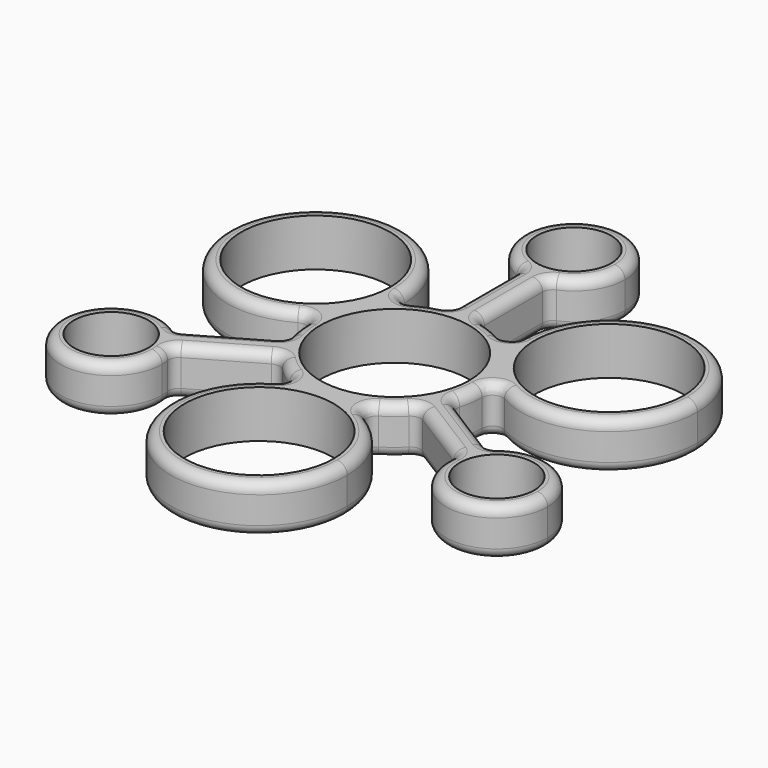
from build123d import *

# Parameters (mm, degrees)
F0_R     = 5.5
F0_R_2   = 11
F1_DEPTH = 7
F2_F1_R  = 1.5
F2_F2_R  = 1.5


with BuildPart() as f1:
    # F0 (on Top) → F1 (new body)
    with BuildSketch(Plane.XY):
        with BuildLine():
            ThreePointArc((2, 25.8452325787), (5.9686681932, 28.5321731949), (7.5, 33.0736487261))
            ThreePointArc((7.5, 33.0736487261), (-4.5414755311, 39.0423169192), (-2, 25.8452325787))
            ThreePointArc((-2, 25.8452325787), (0, 25.5736487261), (2, 25.8452325787))
        make_face()
        with Locations((0, 33.0736487261)):
            Circle(F0_R, mode=Mode.SUBTRACT)
        with BuildLine():
            ThreePointArc((2, 25.8452325787), (0, 25.5736487261), (-2, 25.8452325787))
            Line((-2, 25.8452325787), (-2, 12.8452325787))
            ThreePointArc((-2, 12.8452325787), (0, 13), (2, 12.8452325787))
            Line((2, 12.8452325787), (2, 25.8452325787))
        make_face()
        with BuildLine():
            ThreePointArc((2, 12.8452325787), (0, 13), (-2, 12.8452325787))
            ThreePointArc((-2, 12.8452325787), (-5.7911798985, 11.6388244846), (-9.0399604402, 9.3423292192))
            ThreePointArc((-9.0399604402, 9.3423292192), (-10.3923048454, 6), (-12.6106746544, 3.1576707808))
            ThreePointArc((-12.6106746544, 3.1576707808), (-12.9751076231, -0.8041033323), (-12.1242977306, -4.6905654818))
            ThreePointArc((-12.1242977306, -4.6905654818), (-11.2583302492, -6.5), (-10.1242977306, -8.1546670969))
            ThreePointArc((-10.1242977306, -8.1546670969), (-7.1839277246, -10.8347211523), (-3.5707142143, -12.5))
            ThreePointArc((-3.5707142143, -12.5), (0, -12), (3.5707142143, -12.5))
            ThreePointArc((3.5707142143, -12.5), (7.1839277246, -10.8347211523), (10.1242977306, -8.1546670969))
            ThreePointArc((10.1242977306, -8.1546670969), (11.2590153555, -6.4988132165), (12.1252863318, -4.6880093186))
            ThreePointArc((12.1252863318, -4.6880093186), (12.7794507377, -2.3844577671), (13, 0))
            ThreePointArc((13, 0), (12.9023015487, 1.5907906041), (12.6106746544, 3.1576707808))
            ThreePointArc((12.6106746544, 3.1576707808), (10.3923048454, 6), (9.0399604402, 9.3423292192))
            ThreePointArc((9.0399604402, 9.3423292192), (5.7911798985, 11.6388244846), (2, 12.8452325787))
        make_face()
        Circle(F0_R_2, mode=Mode.SUBTRACT)
        with BuildLine():
            ThreePointArc((-12.6106746544, 3.1576707808), (-10.3923048454, 6), (-9.0399604402, 9.3423292192))
            ThreePointArc((-9.0399604402, 9.3423292192), (-11.2583302492, 6.5), (-12.6106746544, 3.1576707808))
        make_face()
        with BuildLine():
            ThreePointArc((-12.6106746544, 3.1576707808), (-11.2583302492, 6.5), (-9.0399604402, 9.3423292192))
            ThreePointArc((-9.0399604402, 9.3423292192), (-8.7483335459, 10.9092093959), (-8.6506350946, 12.5))
            ThreePointArc((-8.6506350946, 12.5), (-33.6197513051, 17.5734856991), (-12.6106746544, 3.1576707808))
        make_face()
        with Locations((-21.6506350946, 12.5)):
            Circle(F0_R_2, mode=Mode.SUBTRACT)
        with BuildLine():
            ThreePointArc((34.6506350946, 12.5), (20.0598444905, 25.4023015487), (9.0399604402, 9.3423292192))
            ThreePointArc((9.0399604402, 9.3423292192), (11.2583302492, 6.5), (12.6106746544, 3.1576707808))
            ThreePointArc((12.6106746544, 3.1576707808), (26.7241207937, 0.5308837895), (34.6506350946, 12.5))
        make_face()
        with Locations((21.6506350946, 12.5)):
            Circle(F0_R_2, mode=Mode.SUBTRACT)
        with BuildLine():
            ThreePointArc((12.6106746544, 3.1576707808), (11.2583302492, 6.5), (9.0399604402, 9.3423292192))
            ThreePointArc((9.0399604402, 9.3423292192), (10.3923048454, 6), (12.6106746544, 3.1576707808))
        make_face()
        with BuildLine():
            ThreePointArc((-10.1242977306, -8.1546670969), (-11.2583302492, -6.5), (-12.1242977306, -4.6905654818))
            Line((-12.1242977306, -4.6905654818), (-23.3826279798, -11.1905654818))
            ThreePointArc((-23.3826279798, -11.1905654818), (-22.0915188374, -12.743581974), (-21.2616107798, -14.5847977839))
            Line((-21.2616107798, -14.5847977839), (-10.1242977306, -8.1546670969))
        make_face()
        with BuildLine():
            ThreePointArc((-21.2616107798, -14.5847977839), (-22.0915188374, -12.743581974), (-23.3826279798, -11.1905654818))
            ThreePointArc((-23.3826279798, -11.1905654818), (-35.3172804772, -19.7372555098), (-20.9518244327, -16.7180646742))
            ThreePointArc((-20.9518244327, -16.7180646742), (-21.0296750676, -15.6402433525), (-21.2616107798, -14.5847977839))
        make_face()
        with Locations((-28.4518244327, -16.7180646742)):
            Circle(F0_R, mode=Mode.SUBTRACT)
        with BuildLine():
            Line((23.0342028584, -11.5316037925), (12.1252863318, -4.6880093186))
            ThreePointArc((12.1252863318, -4.6880093186), (11.2590153555, -6.4988132165), (10.1242977306, -8.1546670969))
            Line((10.1242977306, -8.1546670969), (21.1366809206, -15.0631702979))
            ThreePointArc((21.1366809206, -15.0631702979), (21.8450992846, -13.1682501977), (23.0342028584, -11.5316037925))
        make_face()
        with BuildLine():
            ThreePointArc((3.5707142143, -12.5), (0, -12), (-3.5707142143, -12.5))
            ThreePointArc((-3.5707142143, -12.5), (0, -13), (3.5707142143, -12.5))
        make_face()
        with BuildLine():
            ThreePointArc((3.5707142143, -12.5), (0, -13), (-3.5707142143, -12.5))
            ThreePointArc((-3.5707142143, -12.5), (-7.8288158496, -35.3783256064), (13, -25))
            ThreePointArc((13, -25), (10.3783256064, -17.1711841504), (3.5707142143, -12.5))
        make_face()
        with Locations((0, -25)):
            Circle(F0_R_2, mode=Mode.SUBTRACT)
        with BuildLine():
            ThreePointArc((35.9518244327, -16.7180646742), (31.2462687596, -9.7581019657), (23.0342028584, -11.5316037925))
            ThreePointArc((23.0342028584, -11.5316037925), (21.8450992846, -13.1682501977), (21.1366809206, -15.0631702979))
            ThreePointArc((21.1366809206, -15.0631702979), (27.6192309969, -24.1717072851), (35.9518244327, -16.7180646742))
        make_face()
        with Locations((28.4518244327, -16.7180646742)):
            Circle(F0_R, mode=Mode.SUBTRACT)
    extrude(amount=F1_DEPTH)

    # F2: fillet of radius 1.5 on 42 edges, made by hand

    # F2_f1
    f2_f1_edges = [f1.edges().sort_by_distance(p)[0] for p in [
        (2, 25.8452325787, 3.5),
        (-2, 25.8452325787, 3.5),
        (12.6106746544, 3.1576707808, 3.5),
        (9.0399604402, 9.3423292192, 3.5),
        (21.1366809206, -15.0631702979, 3.5),
        (23.0342028584, -11.5316037925, 3.5),
        (-3.5707142143, -12.5, 3.5),
        (3.5707142143, -12.5, 3.5),
        (-9.0399604402, 9.3423292192, 3.5),
        (-12.6106746544, 3.1576707808, 3.5),
        (-23.3826279798, -11.1905654818, 3.5),
        (-21.2616107798, -14.5847977839, 3.5),
        (-2, 12.8452325787, 3.5),
        (2, 12.8452325787, 3.5),
        (-12.1242977306, -4.6905654818, 3.5),
        (-10.1242977306, -8.1546670969, 3.5),
        (10.1242977306, -8.1546670969, 3.5),
        (12.1252863318, -4.6880093186, 3.5),
    ]]
    fillet(f2_f1_edges, radius=F2_F1_R)

    # F2_f2
    f2_f2_edges = [f1.edges().sort_by_distance(p)[0] for p in [
        (32.9089653438, 19, 0),
        (32.9089653438, 19, 7),
        (0, -38, 0),
        (0, -38, 7),
        (-32.9089653438, 19, 0),
        (-32.9089653438, 19, 7),
        (-7.9010829335, 11.3149229243, 7),
        (-13.7495521611, 1.1850770757, 7),
        (-7.9010829335, 11.3149229243, 0),
        (-13.7495521611, 1.1850770757, 0),
        (-5.8484692276, -12.5, 7),
        (5.8484692276, -12.5, 7),
        (-5.8484692276, -12.5, 0),
        (5.8484692276, -12.5, 0),
        (13.7495521611, 1.1850770757, 7),
        (7.9010829335, 11.3149229243, 7),
        (13.7495521611, 1.1850770757, 0),
        (7.9010829335, 11.3149229243, 0),
    ]]
    fillet(f2_f2_edges, radius=F2_F2_R)


solid = f1.part
